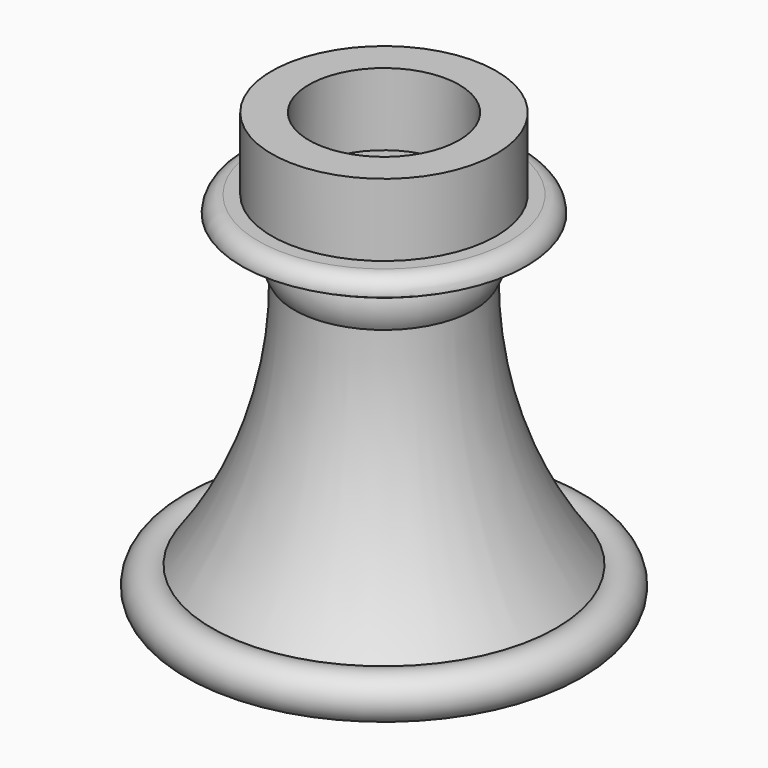
from build123d import *

# Parameters (mm, degrees)
F2_R     = 10.5023561171
F3_DEPTH = 2.032
F4_R     = 1.2264204897
F6_R     = 8.280415088
F6_R_2   = 5.5395009723
F7_DEPTH = 5.334


# Not quite as in the source:
# - a fillet or chamfer that OpenCascade refuses, or shapes differently, is made with other operations: its cross-section is extruded or revolved along the edge and cut away or added


with BuildPart() as f1:
    # F0 (on Front) → F1 (revolve)
    with BuildSketch(Plane.XZ):
        with BuildLine():
            Line((0, 24.7002821416), (0, 0))
            Line((0, 0), (12.7, 0))
            ThreePointArc((12.7, 0), (15.1592770153, 1.3591062743), (12.7, 2.7182125486))
            ThreePointArc((12.7, 2.7182125486), (8.1323573281, 11.5574154189), (6.618256215, 21.3911514729))
            ThreePointArc((6.618256215, 21.3911514729), (7.1000680202, 23.0457168072), (6.618256215, 24.7002821416))
            Line((6.618256215, 24.7002821416), (0, 24.7002821416))
        make_face()
    revolve(axis=Axis((0, 0, 12.3501410708), (0, 0, -1)))

    # F2 (on face) → F3 (join)
    with BuildSketch(Plane.XY.offset(24.7002821416)):
        Circle(F2_R)
    extrude(amount=F3_DEPTH)

    # F4
    f4_edges = [f1.edges().sort_by_distance(p)[0] for p in [
        (-10.502356, 0, 26.732282),
    ]]
    fillet(f4_edges, radius=F4_R)

    # F5: fillet of radius 5.5188922036 on 1 edges, made by hand

    # F5_s1 → F5_t2 (revolve, cut)
    with BuildSketch(Plane.XZ):
        with BuildLine():
            ThreePointArc((10.5023561171, 25.5058616519), (9.1222760715, 24.9054922023), (7.631318916, 24.7002821416))
            Line((7.631318916, 24.7002821416), (7.631318916, 24.5899042975))
            Line((7.631318916, 24.5899042975), (10.5023561171, 24.5899042975))
            Line((10.5023561171, 24.5899042975), (10.6127339612, 24.7002821416))
            ThreePointArc((10.6127339612, 24.7002821416), (10.6127339612, 25.1030718967), (10.5597768612, 25.411595398))
            Line((10.5597768612, 25.411595398), (10.5023561171, 25.5058616519))
        make_face()
    revolve(axis=Axis((0, 0, 24.7002821416), (0, 0, 1)), mode=Mode.SUBTRACT)

    # F6 (on face) → F7 (join)
    with BuildSketch(Plane.XY.offset(26.7322821416)):
        Circle(F6_R)
        Circle(F6_R_2, mode=Mode.SUBTRACT)
    extrude(amount=F7_DEPTH)


solid = f1.part
